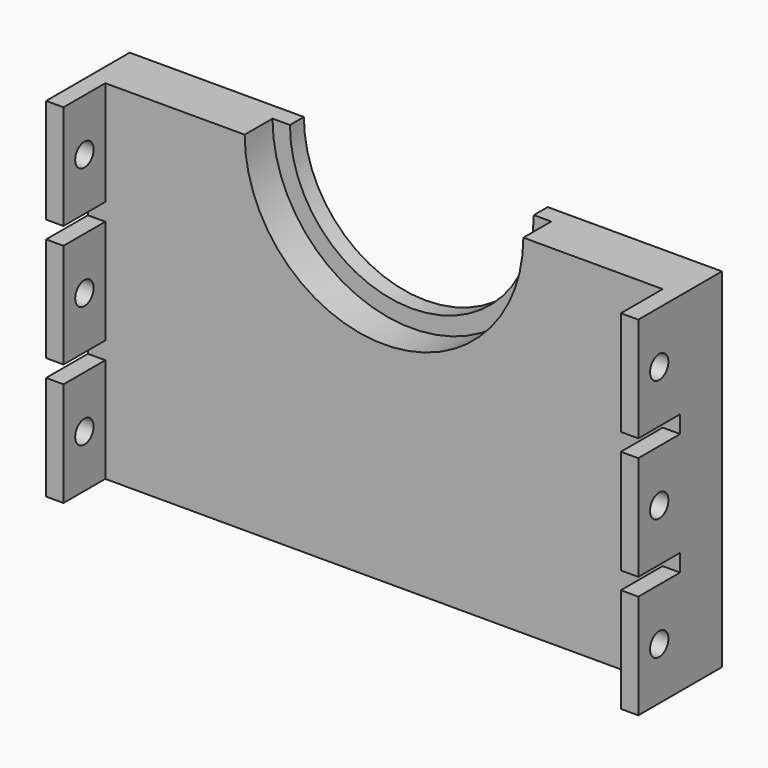
from build123d import *

# Parameters (mm, degrees)
F1_DEPTH = 10
F3_DEPTH = 5
F4_W     = 15
F4_H     = 30
F5_DEPTH = 5
F6_D     = 6.6
F6_DEPTH = 14.25
F6_TIP   = 1.9828400428


# Not quite as in the source:
# - a pattern or mirror of a feature is missing from the dataset's text; its kind, count and spacing are read off the source's solid


with BuildPart() as f1:
    # F0 (on Front) → F1 (new body)
    with BuildSketch(Plane.XZ):
        with BuildLine():
            ThreePointArc((40, 40), (0, 0), (-40, 40))
            Line((-40, 40), (-85, 40))
            Line((-85, 40), (-85, -60))
            Line((-85, -60), (85, -60))
            Line((85, -60), (85, 40))
            Line((85, 40), (40, 40))
        make_face()
    extrude(amount=F1_DEPTH)

    # F2 (on face) → F3 (join)
    with BuildSketch(Plane(origin=(0, 0, 0), x_dir=(-1, 0, 0), z_dir=(0, 1, 0))):
        with BuildLine():
            ThreePointArc((40, 40), (0, 0), (-40, 40))
            Line((-40, 40), (-85, 40))
            Line((-85, 40), (-85, -60))
            Line((-85, -60), (85, -60))
            Line((85, -60), (85, 40))
            Line((85, 40), (40, 40))
        make_face()
        with BuildLine():
            ThreePointArc((35, 40), (0, 5), (-35, 40))
            Line((-35, 40), (-40, 40))
            ThreePointArc((-40, 40), (0, 0), (40, 40))
            Line((40, 40), (35, 40))
        make_face()
    extrude(amount=F3_DEPTH)

    # F4 (on face) → F5 (join)
    with BuildSketch(Plane.YZ.offset(85)):
        with Locations((-17.5, -45)):
            Rectangle(F4_W, F4_H)
        with Locations((-17.5, -10)):
            Rectangle(F4_W, F4_H)
        with Locations((-17.5, 25)):
            Rectangle(F4_W, F4_H)
    f5 = extrude(amount=-F5_DEPTH)

    # F5_copies: F5 across plane
    add(f5.mirror(Plane(origin=(0, 0, 0), x_dir=(0, 0, -1), z_dir=(-1, 0, 0))))

    # F6
    with Locations(Plane.YZ.offset(85)):
        with Locations((-17.5, 25), (-17.5, -10), (-17.5, -45)):
            f6 = Hole(F6_D / 2, depth=F6_DEPTH)
            with Locations((0, 0, -(F6_DEPTH + F6_TIP / 2))):  # 118° drill point
                Cone(0, F6_D / 2, F6_TIP, mode=Mode.SUBTRACT)

    # F6_copies: F6 across plane
    add(f6.mirror(Plane(origin=(0, 0, 0), x_dir=(0, 0, -1), z_dir=(-1, 0, 0))), mode=Mode.SUBTRACT)


solid = f1.part
